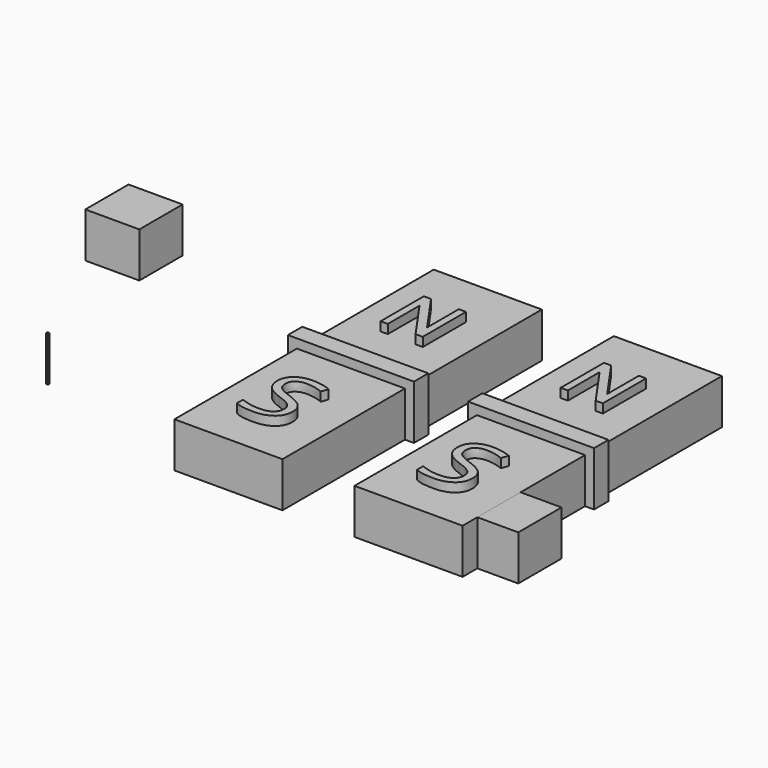
from build123d import *

# Parameters (mm, degrees)
F0_W           = 60
F0_H           = 180
F1_DEPTH       = 25
F2_W           = 1
F2_H           = 1
F3_DEPTH       = 25
F4_W           = 30
F4_H           = 30
F5_DEPTH       = 25
F7_DEPTH       = 5
F8_TEXT_SIZE   = 53.024026512
F9_DEPTH       = 5
F11_DEPTH      = 5
F11_DEPTH_BACK = 25


# Not quite as in the source:
# - Text() gives the source's letters only with a copy of the font that has no kerning and outlines rounded to 1/6400 em; it was checked with that copy


with BuildPart() as f1:
    # F0 (on Top) → F1 (new body)
    with BuildSketch(Plane.XY):
        with Locations((-5.0263749436, -0.4755560953)):
            Rectangle(F0_W, F0_H)
    extrude(amount=F1_DEPTH)

    # F6 (on face) → F7 (join)
    with BuildSketch(Plane.XY.offset(25)):
        Polygon((-16.7286578639, 44.7622219523), (-16.7286578639, 29.7622219523), (-12.7286578639, 29.7622219523), (-12.7286578639, 51.7622219523), (-5.0263749436, 40.7622219523), (2.6759079768, 29.7622219523), (6.6759079768, 29.7622219523), (6.6759079768, 44.7622219523), (6.6759079768, 59.7622219523), (2.6759079768, 59.7622219523), (2.6759079768, 37.7622219523), (-5.0263749436, 48.7622219523), (-12.7286578639, 59.7622219523), (-16.7286578639, 59.7622219523), align=None)
    extrude(amount=F7_DEPTH)

    # F8 (on face) → F9 (join)
    with BuildSketch(Plane.XY.offset(25)):
        with Locations((-20.0263749436, -70.4755560953)):
            Text('S', F8_TEXT_SIZE, font='Open Sans', text_align=(TextAlign.LEFT, TextAlign.BOTTOM))
    extrude(amount=F9_DEPTH)

    # F10 (on face) → F11 (join, two sides)
    with BuildSketch(Plane.XY.offset(25)) as f11_sk:
        Polygon((24.9736250564, -5.4757087717), (24.9736250564, -0.4755560953), (-35.0263749436, 0), (-35.0263749436, -5.4757087717), (-5.0263749436, -5.4757087717), align=None)
        Polygon((-35.0263749436, 0), (24.9736250564, -0.4755560953), (24.9736250564, 4.5242912283), (-5.0263749436, 4.5242912283), (-35.0263749436, 4.5242912283), align=None)
        Polygon((24.9736250564, 4.5242912283), (24.9736250564, -0.4755560953), (24.9736250564, -5.4757087717), (29.9736250564, -5.4757087717), (29.9736250564, 4.5242912283), align=None)
        Polygon((-35.0263749436, -5.4757087717), (-35.0263749436, 0), (-35.0263749436, 4.5242912283), (-40.0263749436, 4.5242912283), (-40.0263749436, -5.4757087717), align=None)
    extrude(amount=F11_DEPTH)
    extrude(f11_sk.sketch, amount=-F11_DEPTH_BACK)


with BuildPart() as f3:
    # F2 (on Top) → F3 (new body)
    with BuildSketch(Plane.XY):
        with Locations((-128.5935565829, -61.4509395935)):
            Rectangle(F2_W, F2_H)
    extrude(amount=F3_DEPTH)


with BuildPart() as f5:
    # F4 (on Top) → F5 (new body)
    with BuildSketch(Plane.XY):
        with Locations((-173.2785601946, 54.2563074516)):
            Rectangle(F4_W, F4_H)
    extrude(amount=F5_DEPTH)


with BuildPart() as f5b:
    # F4 (on Top) → F5, piece 2 (new body)
    with BuildSketch(Plane.XY):
        with Locations((132.7215333315, -65.2437285949)):
            Rectangle(F4_W, F4_H)
    extrude(amount=F5_DEPTH)


with BuildPart() as f12_1:
    # F12: copy of F1
    add(f1.part.moved(Location((100, 0, 0))))


solid = Compound([f1.part, f3.part, f5.part, f5b.part, f12_1.part])
